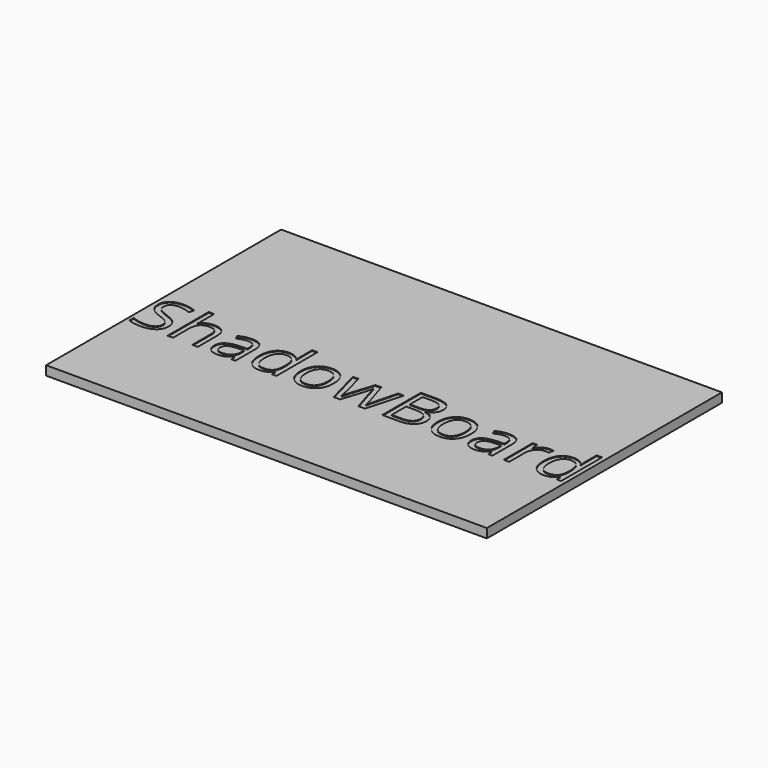
from build123d import *

# Parameters (mm, degrees)
F0_W         = 914.4
F0_H         = 609.6
F1_DEPTH     = 19.05
F2_TEXT_SIZE = 140.2117974028
F3_DEPTH     = 1.5875


# Not quite as in the source:
# - Text() gives the source's letters only with a copy of the font that has no kerning and outlines rounded to 1/6400 em; it was checked with that copy


with BuildPart() as f1:
    # F0 (on Top) → F1 (new body)
    with BuildSketch(Plane.XY):
        Rectangle(F0_W, F0_H)
    extrude(amount=F1_DEPTH)

    # F2 (on face) → F3 (cut)
    with BuildSketch(Plane.XY.offset(19.05)):
        with Locations((-457.2, -100.95249413)):
            Text('ShadowBoard', F2_TEXT_SIZE, font='Open Sans', text_align=(TextAlign.LEFT, TextAlign.BOTTOM))
    extrude(amount=-F3_DEPTH, mode=Mode.SUBTRACT)


solid = f1.part
